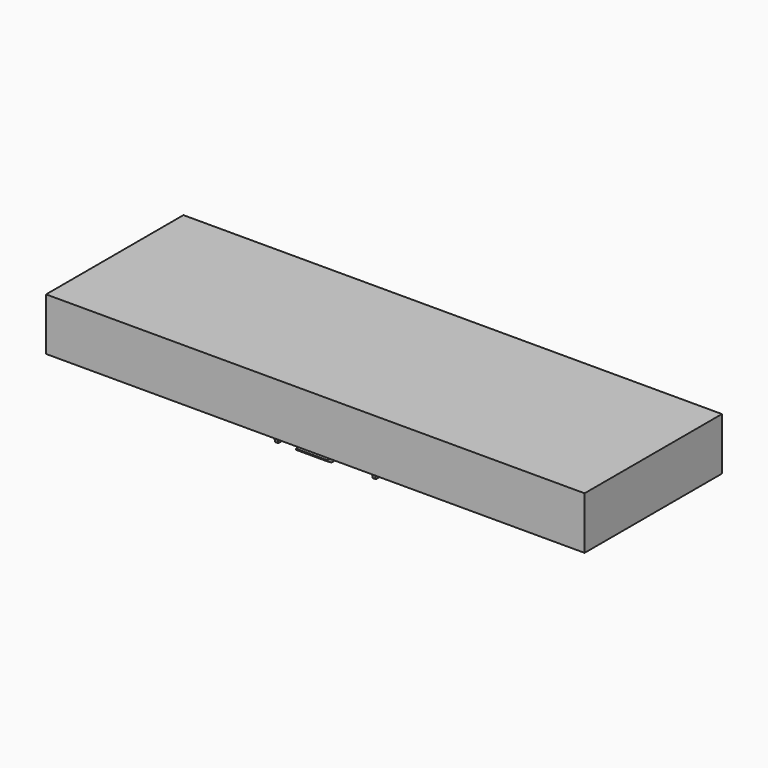
from build123d import *

# Parameters (mm, degrees)
F11_DEPTH       = 2
F12_W           = 1.5
F12_H           = 7.2
F13_DEPTH       = 6
F14_R           = 4.25
F15_DEPTH       = 3
F16_R           = 8
F17_DEPTH       = 0.3
F19_D           = 4.3
F19_CSINK_D     = 8.7
F19_CSINK_ANGLE = 90
F20_SIZE2       = 1.5
F20_SIZE        = 2.5
F21_SIZE2       = 3.99999
F21_SIZE        = 0.99999
F21_2_SIZE2     = 3.99999
F21_2_SIZE      = 0.99999
F22_SIZE2       = 3.99999
F22_SIZE        = 0.99999
F24_W           = 256.5929293633
F24_H           = 81.7903461866
F25_DEPTH       = 25


# Not quite as in the source:
# - a fillet or chamfer is up to 0.001 mm smaller than in the source, because OpenCascade refuses the exact size


with BuildPart() as f11:
    # F10 (on Top) → F11 (new body, through all)
    with BuildSketch(Plane.XY):
        Polygon((-24, 0), (-7.5, 0), (-7.5, -5), (0, -5), (0, 24), (-1.5, 24), (-1.5, 22), (-24, 22), (-24, 12.5), (-26, 12.5), (-26, 9.5), (-24, 9.5), align=None)
    extrude(amount=-F11_DEPTH)

    # F12 (on Top) → F13 (join, through all)
    with BuildSketch(Plane.XY):
        with Locations((-23.25, 5.9)):
            Rectangle(F12_W, F12_H)
        with Locations((-23.25, 16.1)):
            Rectangle(F12_W, F12_H)
    extrude(amount=-F13_DEPTH)

    # F14 (on Top) → F15 (join, through all)
    with BuildSketch(Plane.XY):
        with Locations((-12, 11)):
            Circle(F14_R)
    extrude(amount=-F15_DEPTH)

    # F16 (on Top) → F17 (join, through all)
    with BuildSketch(Plane.XY):
        with Locations((-12, 11)):
            Circle(F16_R)
    extrude(amount=F17_DEPTH)

    # F19 (through all)
    with Locations(Plane.XY.offset(0.3)):
        with Locations((-12, 11)):
            CounterSinkHole(F19_D / 2, F19_CSINK_D / 2, counter_sink_angle=F19_CSINK_ANGLE)

    # F20
    f20_edges = [f11.edges().sort_by_distance(p)[0] for p in [
        (-3.75, -5, -2),
    ]]
    f20_side = f11.faces().sort_by_distance((-23.610513, 1.15, -2))[0]
    chamfer(f20_edges, length=F20_SIZE, length2=F20_SIZE2, reference=f20_side)

    # F21 (size 1 and 4 in the source; OpenCascade refuses exactly that, so slightly less here)
    f21_edges = [f11.edges().sort_by_distance(p)[0] for p in [
        (-23.25, 2.3, -6),
        (-23.25, 9.5, -6),
    ]]
    f21_side = f11.faces().sort_by_distance((-23.25, 5.9, -6))[0]
    chamfer(f21_edges, length=F21_SIZE, length2=F21_SIZE2, reference=f21_side)

    # F21#2 (size 1 and 4 in the source; OpenCascade refuses exactly that, so slightly less here)
    f21_2_edges = [f11.edges().sort_by_distance(p)[0] for p in [
        (-23.25, 12.5, -6),
    ]]
    f21_2_side = f11.faces().sort_by_distance((-23.25, 16.1, -6))[0]
    chamfer(f21_2_edges, length=F21_2_SIZE, length2=F21_2_SIZE2, reference=f21_2_side)

    # F22 (size 1 and 4 in the source; OpenCascade refuses exactly that, so slightly less here)
    f22_edges = [f11.edges().sort_by_distance(p)[0] for p in [
        (-23.25, 19.7, -6),
    ]]
    f22_side = f11.faces().sort_by_distance((-23.25, 16.599995, -6))[0]
    chamfer(f22_edges, length=F22_SIZE, length2=F22_SIZE2, reference=f22_side)

    # F23: F11 across plane


with BuildPart() as f11_1:
    add(f11.part)
    add(f11.part.mirror(Plane.YZ))


with BuildPart() as f25:
    # F24 (on offset) → F25 (new body)
    with BuildSketch(Plane.XY.offset(0.3)):
        with Locations((0.9540170431, 36.935655633)):
            Rectangle(F24_W, F24_H)
    extrude(amount=F25_DEPTH)


solid = Compound([f11_1.part, f25.part])
